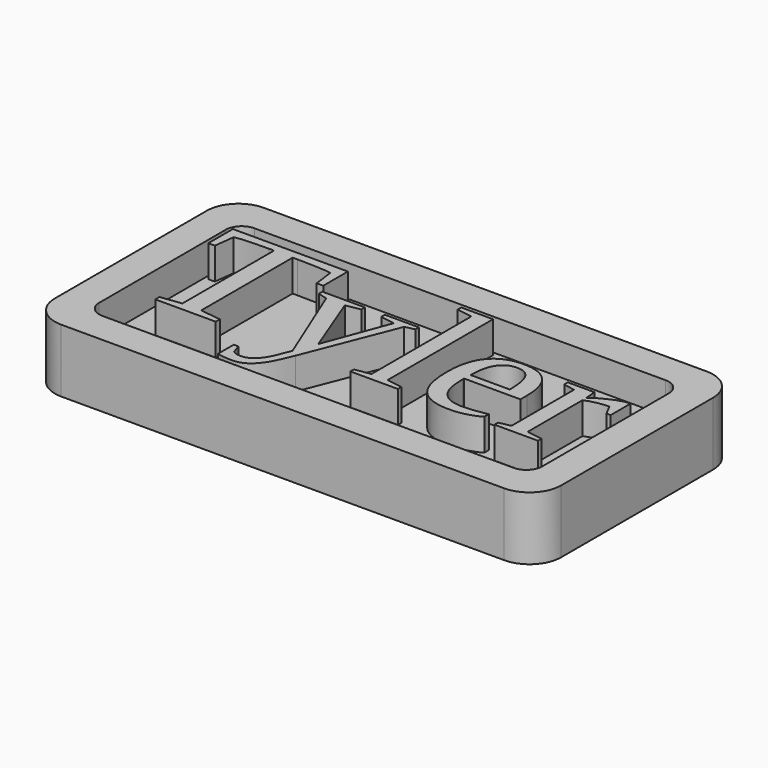
from build123d import *

# Parameters (mm, degrees)
F1_DEPTH     = 6.35
F3_DEPTH     = 3.175
F4_TEXT_SIZE = 20.0295712173
F5_DEPTH     = 3.175


# Not quite as in the source:
# - Text() gives the source's letters only with a copy of the font that has no kerning and outlines rounded to 1/6400 em; it was checked with that copy


with BuildPart() as f1:
    # F0 (on Top) → F1 (new body)
    with BuildSketch(Plane.XY):
        with BuildLine():
            Line((47.625, 25.4), (3.175, 25.4))
            ThreePointArc((3.175, 25.4), (0.9299359697, 24.4700640303), (0, 22.225))
            Line((0, 22.225), (0, 3.175))
            ThreePointArc((0, 3.175), (0.9299359697, 0.9299359697), (3.175, 0))
            Line((3.175, 0), (47.625, 0))
            ThreePointArc((47.625, 0), (49.8700640303, 0.9299359697), (50.8, 3.175))
            Line((50.8, 3.175), (50.8, 22.225))
            ThreePointArc((50.8, 22.225), (49.8700640303, 24.4700640303), (47.625, 25.4))
        make_face()
    extrude(amount=F1_DEPTH)

    # F2 (on face) → F3 (cut)
    with BuildSketch(Plane.XY.offset(6.35)):
        with BuildLine():
            Line((46.0375, 22.225), (4.7625, 22.225))
            ThreePointArc((4.7625, 22.225), (3.6399679849, 21.7600320151), (3.175, 20.6375))
            Line((3.175, 20.6375), (3.175, 4.7625))
            ThreePointArc((3.175, 4.7625), (3.6399679849, 3.6399679849), (4.7625, 3.175))
            Line((4.7625, 3.175), (46.0375, 3.175))
            ThreePointArc((46.0375, 3.175), (47.1600320151, 3.6399679849), (47.625, 4.7625))
            Line((47.625, 4.7625), (47.625, 20.6375))
            ThreePointArc((47.625, 20.6375), (47.1600320151, 21.7600320151), (46.0375, 22.225))
        make_face()
    extrude(amount=-F3_DEPTH, mode=Mode.SUBTRACT)

    # F4 (on face) → F5 (join)
    with BuildSketch(Plane.XY.offset(3.175)):
        with Locations((3.175, 7.9570829869)):
            Text('Tyler', F4_TEXT_SIZE, font='Tinos', text_align=(TextAlign.LEFT, TextAlign.BOTTOM))
    extrude(amount=F5_DEPTH)


solid = f1.part
